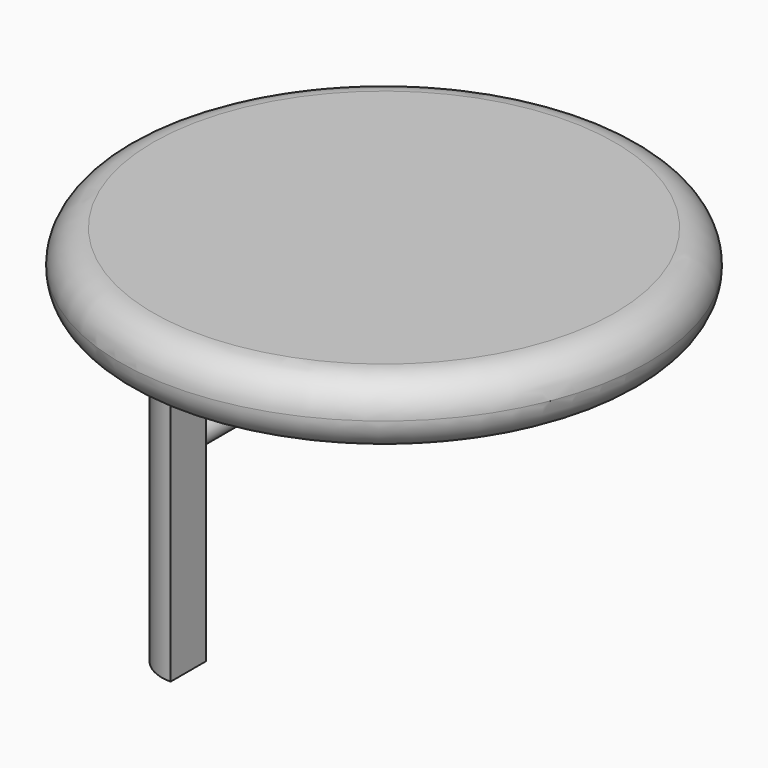
from build123d import *

# Parameters (mm, degrees)
F0_R     = 304.8
F1_DEPTH = 76.2
F2_R     = 38.09999
F3_W     = 50.8
F3_H     = 431.8
F4_DEPTH = 50.8
F5_R     = 50.79999
F7_DEPTH = 304.8


# Not quite as in the source:
# - a fillet or chamfer is up to 0.001 mm smaller than in the source, because OpenCascade refuses the exact size


with BuildPart() as f1:
    # F0 (on Top) → F1 (new body)
    with BuildSketch(Plane.XY):
        Circle(F0_R)
    extrude(amount=F1_DEPTH)

    # F2 (radius 38.1 in the source; OpenCascade refuses exactly that, so slightly less here)
    f2_edges = [f1.edges().sort_by_distance(p)[0] for p in [
        (-304.8, 0, 76.2),
        (-304.8, 0, 0),
    ]]
    fillet(f2_edges, radius=F2_R)


with BuildPart() as f4:
    # F3 (on Front) → F4 (new body)
    with BuildSketch(Plane.XZ):
        with Locations((-231.2447311898, -215.9)):
            Rectangle(F3_W, F3_H)
    extrude(amount=F4_DEPTH)

    # F5 (radius 50.8 in the source; OpenCascade refuses exactly that, so slightly less here)
    f5_edges = [f4.edges().sort_by_distance(p)[0] for p in [
        (-256.644731, -50.8, -215.9),
    ]]
    fillet(f5_edges, radius=F5_R)

    # F6 (on face) → F7 (join)
    with BuildSketch(Plane(origin=(0, 0, 0), x_dir=(-1, 0, 0), z_dir=(0, 1, 0))):
        with BuildLine():
            ThreePointArc((243.9447311898, -215.9), (240.2249873109, -206.9197438789), (231.2447311898, -203.2))
            Line((231.2447311898, -203.2), (231.2447311898, -228.6))
            ThreePointArc((231.2447311898, -228.6), (240.2249873109, -224.8802561211), (243.9447311898, -215.9))
        make_face()
        with BuildLine():
            Line((231.2447311898, -228.6), (231.2447311898, -203.2))
            ThreePointArc((231.2447311898, -203.2), (218.5447311898, -215.9), (231.2447311898, -228.6))
        make_face()
    extrude(amount=F7_DEPTH)


solid = Compound([f1.part, f4.part])
